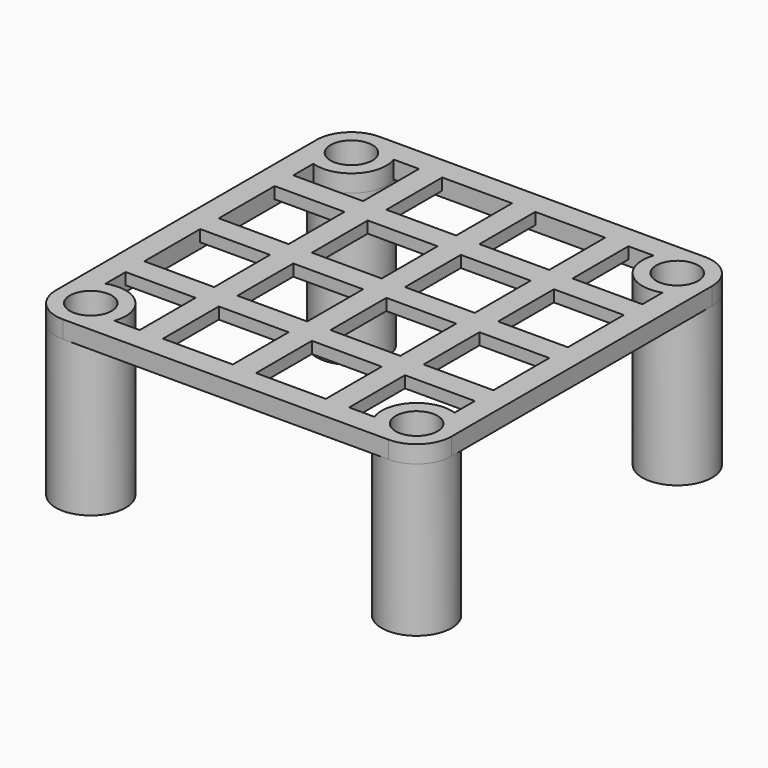
from build123d import *
from build123d import SkipClean  # not in build123d's __all__

# Parameters (mm, degrees)
F0_R     = 3
F0_R_2   = 1.8
F1_DEPTH = 13
F2_R     = 1.8
F3_DEPTH = 1.5
F4_W     = 6
F4_H     = 6
F5_DEPTH = 1


with BuildPart() as f1:
    # F0 (on Top) → F1 (new body)
    with BuildSketch(Plane.XY):
        with Locations((-14, 14)):
            Circle(F0_R)
        with Locations((-14, 14)):
            Circle(F0_R_2, mode=Mode.SUBTRACT)
    extrude(amount=F1_DEPTH)



with BuildPart() as f1b:
    # F0 (on Top) → F1, piece 2 (new body)
    with BuildSketch(Plane.XY):
        with Locations((-14, -14)):
            Circle(F0_R)
        with Locations((-14, -14)):
            Circle(F0_R_2, mode=Mode.SUBTRACT)
    extrude(amount=F1_DEPTH)


with BuildPart() as f1c:
    # F0 (on Top) → F1, piece 3 (new body)
    with BuildSketch(Plane.XY):
        with Locations((14, -14)):
            Circle(F0_R)
        with Locations((14, -14)):
            Circle(F0_R_2, mode=Mode.SUBTRACT)
    extrude(amount=F1_DEPTH)


with BuildPart() as f1d:
    # F0 (on Top) → F1, piece 4 (new body)
    with BuildSketch(Plane.XY):
        with Locations((14, 14)):
            Circle(F0_R)
        with Locations((14, 14)):
            Circle(F0_R_2, mode=Mode.SUBTRACT)
    extrude(amount=F1_DEPTH)


with BuildPart() as f1_1:
    add(f1.part, clean=False)

    with SkipClean():  # cleaning this boolean's faces spoils the solid; the shape is the same uncleaned
        add(f1b.part)  # F3 merges F1b

    with SkipClean():  # cleaning this boolean's faces spoils the solid; the shape is the same uncleaned
        add(f1c.part)  # F3 merges F1c

    with SkipClean():  # cleaning this boolean's faces spoils the solid; the shape is the same uncleaned
        add(f1d.part)  # F3 merges F1d
    # F2 (on face) → F3 (join)
    with BuildSketch(Plane.XY.offset(13)):
        with BuildLine():
            Line((14, 17), (-14, 17))
            ThreePointArc((-14, 17), (-16.1213203436, 16.1213203436), (-17, 14))
            Line((-17, 14), (-17, -14))
            ThreePointArc((-17, -14), (-16.1213203436, -16.1213203436), (-14, -17))
            Line((-14, -17), (14, -17))
            ThreePointArc((14, -17), (16.1213203436, -16.1213203436), (17, -14))
            Line((17, -14), (17, 14))
            ThreePointArc((17, 14), (16.1213203436, 16.1213203436), (14, 17))
        make_face()
        with Locations((-14, -14)):
            Circle(F2_R, mode=Mode.SUBTRACT)
        with Locations((14, -14)):
            Circle(F2_R, mode=Mode.SUBTRACT)
        with Locations((-14, 14)):
            Circle(F2_R, mode=Mode.SUBTRACT)
        with BuildLine():
            Line((-15, -11.1715728753), (-15, 11.1715728753))
            ThreePointArc((-15, 11.1715728753), (-11.8786796564, 11.8786796564), (-11.1715728753, 15))
            Line((-11.1715728753, 15), (11.1715728753, 15))
            ThreePointArc((11.1715728753, 15), (11.8786796564, 11.8786796564), (15, 11.1715728753))
            Line((15, 11.1715728753), (15, -11.1715728753))
            ThreePointArc((15, -11.1715728753), (11.8786796564, -11.8786796564), (11.1715728753, -15))
            Line((11.1715728753, -15), (-11.1715728753, -15))
            ThreePointArc((-11.1715728753, -15), (-11.8786796564, -11.8786796564), (-15, -11.1715728753))
        make_face(mode=Mode.SUBTRACT)
        with Locations((14, 14)):
            Circle(F2_R, mode=Mode.SUBTRACT)
    with SkipClean():  # cleaning this boolean's faces spoils the solid; the shape is the same uncleaned
        extrude(amount=F3_DEPTH)

    # F4 (on face) → F5 (join)
    with BuildSketch(Plane.XY.offset(14.5)):
        Polygon((1, 15), (-1, 15), (-1, 9), (-7, 9), (-7, 15), (-9, 15), (-9, 9), (-15, 9), (-15, 7), (-9, 7), (-9, 1), (-15, 1), (-15, -1), (-9, -1), (-9, -7), (-15, -7), (-15, -9), (-9, -9), (-9, -15), (-7, -15), (-7, -9), (-1, -9), (-1, -15), (1, -15), (1, -9), (7, -9), (7, -15), (9, -15), (9, -9), (15, -9), (15, -7), (9, -7), (9, -1), (15, -1), (15, 1), (9, 1), (9, 7), (15, 7), (15, 9), (9, 9), (9, 15), (7, 15), (7, 9), (1, 9), align=None)
        with Locations((-4, -4)):
            Rectangle(F4_W, F4_H, mode=Mode.SUBTRACT)
        with Locations((4, -4)):
            Rectangle(F4_W, F4_H, mode=Mode.SUBTRACT)
        with Locations((-4, 4)):
            Rectangle(F4_W, F4_H, mode=Mode.SUBTRACT)
        with Locations((4, 4)):
            Rectangle(F4_W, F4_H, mode=Mode.SUBTRACT)
    extrude(amount=-F5_DEPTH)


solid = f1_1.part
